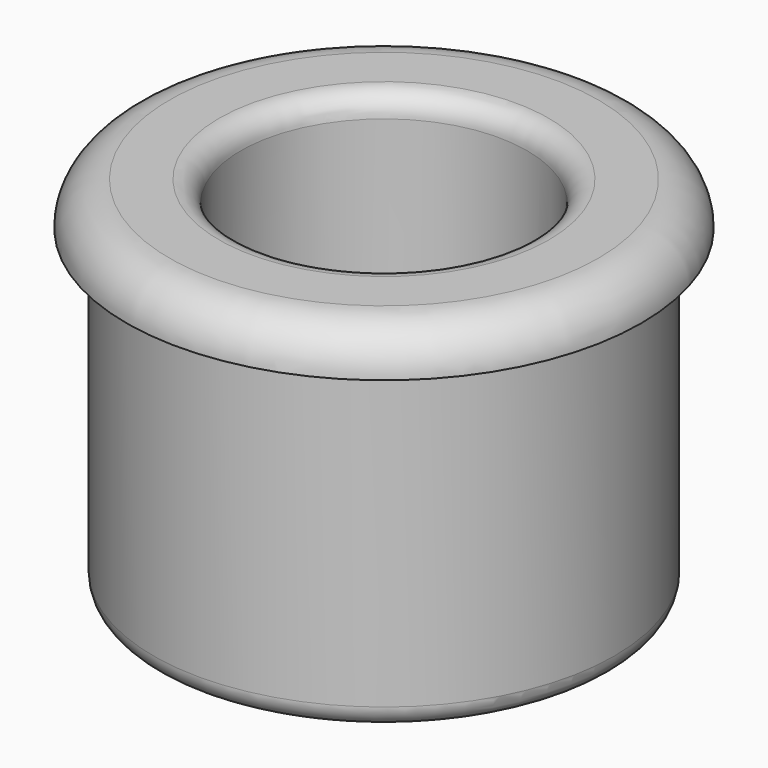
from build123d import *

# Parameters (mm, degrees)
F0_R     = 27.178
F0_R_2   = 16.891
F1_DEPTH = 38.1
F2_R     = 30.353
F2_R_2   = 27.178
F2_R_3   = 16.891
F3_DEPTH = 5.08
F5_D     = 10.0838
F5_DEPTH = 30.354
F6_R     = 2.54
F7_R     = 5.07999


# Not quite as in the source:
# - a fillet or chamfer is up to 0.001 mm smaller than in the source, because OpenCascade refuses the exact size


with BuildPart() as f1:
    # F0 (on Top) → F1 (new body)
    with BuildSketch(Plane.XY):
        Circle(F0_R)
        Circle(F0_R_2, mode=Mode.SUBTRACT)
    extrude(amount=F1_DEPTH)

    # F2 (on face) → F3 (join)
    with BuildSketch(Plane.XY.offset(38.1)):
        Circle(F2_R)
        Circle(F2_R_2, mode=Mode.SUBTRACT)
        Circle(F2_R_2)
        Circle(F2_R_3, mode=Mode.SUBTRACT)
    extrude(amount=F3_DEPTH)

    # F5 (through all, one way)
    with BuildSketch(Plane.XZ):
        with Locations((0, 16.51)):
            Circle(F5_D / 2)
    extrude(amount=-F5_DEPTH, mode=Mode.SUBTRACT)

    # F6
    f6_edges = [f1.edges().sort_by_distance(p)[0] for p in [
        (-16.891, 0, 0),
        (-27.178, 0, 0),
        (-16.891, 0, 43.18),
    ]]
    fillet(f6_edges, radius=F6_R)

    # F7 (radius 5.08 in the source; OpenCascade refuses exactly that, so slightly less here)
    f7_edges = [f1.edges().sort_by_distance(p)[0] for p in [
        (-30.353, 0, 43.18),
    ]]
    fillet(f7_edges, radius=F7_R)


solid = f1.part
